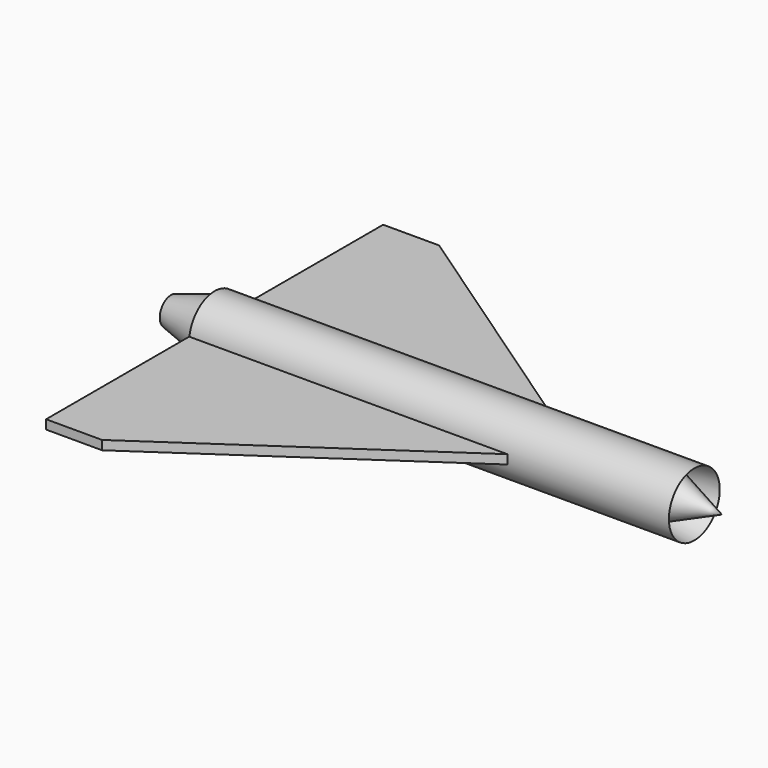
from build123d import *

# Parameters (mm, degrees)
F3_DEPTH      = 1
F3_DEPTH_BACK = 1


with BuildPart() as f1:
    # F0 (on Top) → F1 (revolve)
    with BuildSketch(Plane.XY):
        Polygon((60.1996816695, 19.7308845818), (-60.7725344598, 19.7308845818), (-60.7725344598, 16.6342694638), (-51.2052008978, 13.7744341046), (-51.2052008978, 12.7527546138), (24.6576368012, 12.7527546138), (33.5514515318, 14.7610362619), (41.0273786474, 14.7610362619), (48.503305763, 14.7610362619), align=None)
        Polygon((54.1369915009, 12.7527546138), (41.0273786474, 14.7610362619), (33.5514515318, 14.7610362619), (24.6576368012, 12.7527546138), align=None)
    revolve(axis=Axis((-0.2864263952, 19.7308845818, 0), (1, 0, 0)))


with BuildPart() as f3:
    # F2 (on Top) → F3 (new body, two sides)
    with BuildSketch(Plane.XY) as f3_sk:
        Polygon((-51.2052008978, 65.988779068), (-51.2052008978, 26.7090145499), (18.6587013304, 26.7090145499), (-38.9073677361, 65.988779068), align=None)
    extrude(amount=F3_DEPTH)
    extrude(f3_sk.sketch, amount=-F3_DEPTH_BACK)


with BuildPart() as f3b:
    # F2 (on Top) → F3, piece 2 (new body, two sides)
    with BuildSketch(Plane.XY) as f3_2_sk:
        Polygon((-38.9073677361, -26.5270099044), (18.6587013304, 12.7527546138), (-51.2052008978, 12.7527546138), (-51.2052008978, -26.5270099044), align=None)
    extrude(amount=F3_DEPTH)
    extrude(f3_2_sk.sketch, amount=-F3_DEPTH_BACK)


solid = Compound([f1.part, f3.part, f3b.part])
